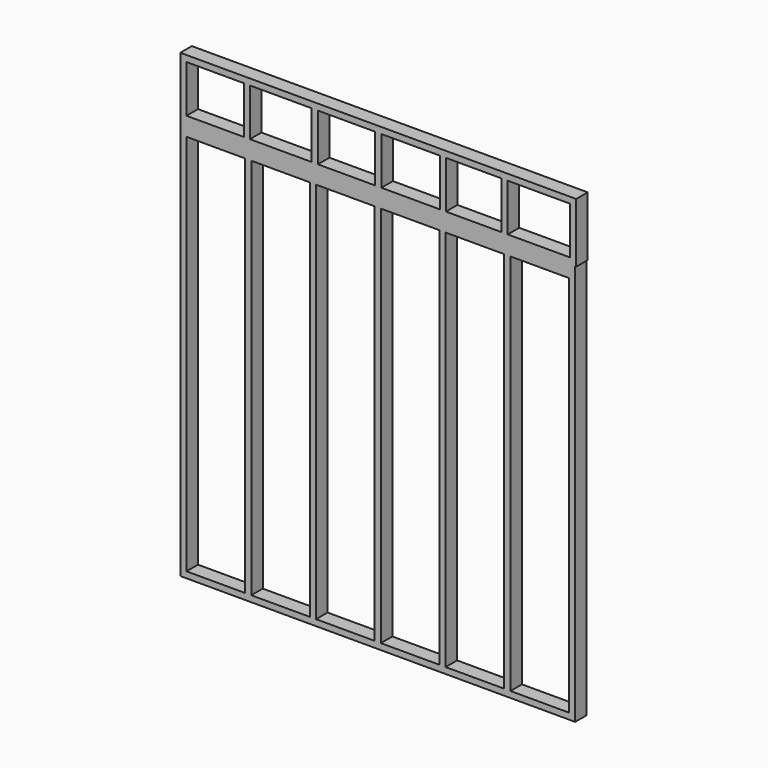
from build123d import *

# Parameters (mm, degrees)
F0_W     = 2438.4
F0_H     = 2438.4
F0_W_2   = 38.1
F0_H_2   = 292.1
F0_H_3   = 2362.2
F0_H_4   = 38.1
F1_DEPTH = 88.9


# Not quite as in the source:
# - a feature names something its author has since deleted; it is built from what else it names


with BuildPart() as f1:
    # F0 (on Front) → F1 (new body)
    with BuildSketch(Plane.XZ):
        with Locations((42.6727382223, -69.3937962841)):
            Rectangle(F0_W, F0_H)
        Polygon((-1138.4272617777, -1250.4937962841), (-1138.4272617777, 1111.7062037159), (-776.4772617777, 1111.7062037159), (-738.3772617777, 1111.7062037159), (-376.4272617777, 1111.7062037159), (-338.3272617777, 1111.7062037159), (23.6227382223, 1111.7062037159), (61.7227382223, 1111.7062037159), (423.6727382223, 1111.7062037159), (461.7727382223, 1111.7062037159), (823.7227382223, 1111.7062037159), (861.8227382223, 1111.7062037159), (1175.4527852575, 1111.7062037159), (1223.7727382223, 1111.7062037159), (1223.7727382223, -1250.4937962841), (861.8227382223, -1250.4937962841), (823.7227382223, -1250.4937962841), (461.7727382223, -1250.4937962841), (423.6727382223, -1250.4937962841), (61.7227382223, -1250.4937962841), (23.6227382223, -1250.4937962841), (-338.3272617777, -1250.4937962841), (-376.4272617777, -1250.4937962841), (-738.3772617777, -1250.4937962841), (-776.4772617777, -1250.4937962841), align=None, mode=Mode.SUBTRACT)
        Polygon((-1176.5272617777, 1556.2062037159), (-1176.5272617777, 1187.9062037159), (1261.8727382223, 1187.9062037159), (1267.9077571224, 1187.9062037159), (1267.9077571224, 1556.2062037159), align=None)
        Polygon((-1138.4272617777, 1226.0062037159), (-1138.4272617777, 1518.1062037159), (-784.7508192062, 1518.1062037159), (-746.6508192062, 1518.1062037159), (-365.0607764721, 1518.1062037159), (-326.9607764721, 1518.1062037159), (27.0738322288, 1518.1062037159), (65.1738322288, 1518.1062037159), (425.5673885345, 1518.1062037159), (463.6673885345, 1518.1062037159), (807.1037530899, 1518.1062037159), (845.2037530899, 1518.1062037159), (1229.8077571224, 1518.1062037159), (1229.8077571224, 1226.0062037159), (845.2037530899, 1226.0062037159), (807.1037530899, 1226.0062037159), (463.6673885345, 1226.0062037159), (425.5673885345, 1226.0062037159), (65.1738322288, 1226.0062037159), (27.0738322288, 1226.0062037159), (-326.9607764721, 1226.0062037159), (-365.0607764721, 1226.0062037159), (-746.6508192062, 1226.0062037159), (-784.7508192062, 1226.0062037159), align=None, mode=Mode.SUBTRACT)
        with Locations((-765.7008192062, 1372.0562037159)):
            Rectangle(F0_W_2, F0_H_2)
        with Locations((442.7227382223, -69.3937962841)):
            Rectangle(F0_W_2, F0_H_3)
        with Locations((842.7727382223, -69.3937962841)):
            Rectangle(F0_W_2, F0_H_3)
        with Locations((42.6727382223, 1168.8562037159)):
            Rectangle(F0_W, F0_H_4)
        with Locations((-346.0107764721, 1372.0562037159)):
            Rectangle(F0_W_2, F0_H_2)
        with Locations((-357.3772617777, -69.3937962841)):
            Rectangle(F0_W_2, F0_H_3)
        with Locations((42.6727382223, -69.3937962841)):
            Rectangle(F0_W_2, F0_H_3)
        with Locations((46.1238322288, 1372.0562037159)):
            Rectangle(F0_W_2, F0_H_2)
        with Locations((-757.4272617777, -69.3937962841)):
            Rectangle(F0_W_2, F0_H_3)
        with Locations((444.6173885345, 1372.0562037159)):
            Rectangle(F0_W_2, F0_H_2)
        with Locations((826.1537530899, 1372.0562037159)):
            Rectangle(F0_W_2, F0_H_2)
    extrude(amount=F1_DEPTH)


solid = f1.part
